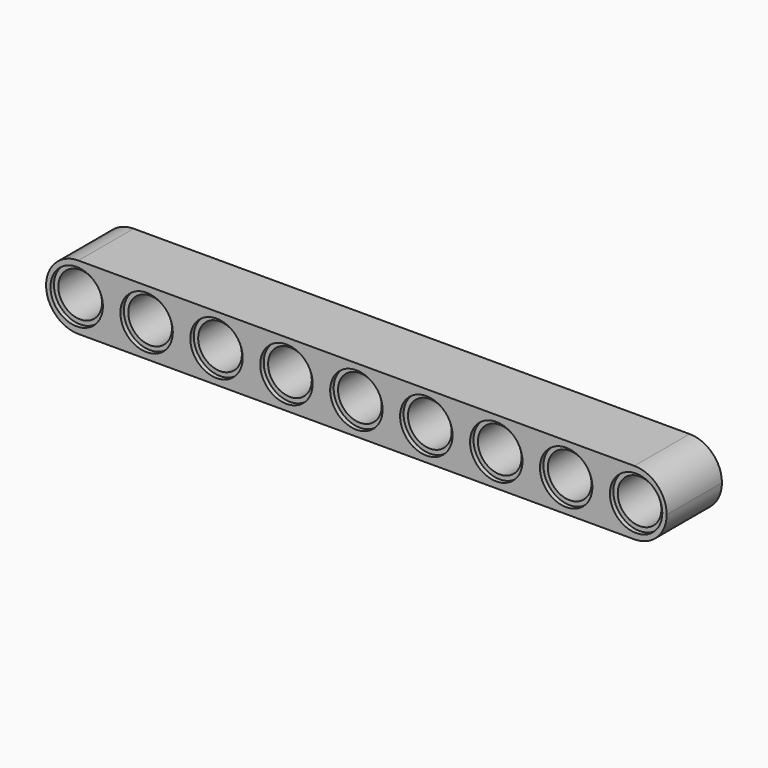
from build123d import *

# Parameters (mm, degrees)
F1_DEPTH = 3.95
F2_DEPTH = 3.45
F3_R     = 3.69999


# Not quite as in the source:
# - a fillet or chamfer is up to 0.001 mm smaller than in the source, because OpenCascade refuses the exact size


with BuildPart() as f1:
    # F0 (on Front) → F1 (new body, symmetric)
    with BuildSketch(Plane.XZ):
        with BuildLine():
            Line((21.3529593349, -11.1881163925), (-49.6470406651, -11.1881163925))
            Line((-49.6470406651, -11.1881163925), (-49.6470406651, -14.8881163925))
            Line((-49.6470406651, -14.8881163925), (-49.1470406651, -14.8881163925))
            ThreePointArc((-49.1470406651, -14.8881163925), (-46.1470406651, -11.8881163925), (-43.1470406651, -14.8881163925))
            Line((-43.1470406651, -14.8881163925), (-41.1470406651, -14.8881163925))
            ThreePointArc((-41.1470406651, -14.8881163925), (-38.1470406651, -11.8881163925), (-35.1470406651, -14.8881163925))
            Line((-35.1470406651, -14.8881163925), (-33.1470406651, -14.8881163925))
            ThreePointArc((-33.1470406651, -14.8881163925), (-30.1470406651, -11.8881163925), (-27.1470406651, -14.8881163925))
            Line((-27.1470406651, -14.8881163925), (-25.1470406651, -14.8881163925))
            ThreePointArc((-25.1470406651, -14.8881163925), (-22.1470406651, -11.8881163925), (-19.1470406651, -14.8881163925))
            Line((-19.1470406651, -14.8881163925), (-17.1470406651, -14.8881163925))
            ThreePointArc((-17.1470406651, -14.8881163925), (-14.1470406651, -11.8881163925), (-11.1470406651, -14.8881163925))
            Line((-11.1470406651, -14.8881163925), (-9.1470406651, -14.8881163925))
            ThreePointArc((-9.1470406651, -14.8881163925), (-6.1470406651, -11.8881163925), (-3.1470406651, -14.8881163925))
            Line((-3.1470406651, -14.8881163925), (-1.1470406651, -14.8881163925))
            ThreePointArc((-1.1470406651, -14.8881163925), (1.8529593349, -11.8881163925), (4.8529593349, -14.8881163925))
            Line((4.8529593349, -14.8881163925), (6.8529593349, -14.8881163925))
            ThreePointArc((6.8529593349, -14.8881163925), (9.8529593349, -11.8881163925), (12.8529593349, -14.8881163925))
            Line((12.8529593349, -14.8881163925), (14.8529593349, -14.8881163925))
            ThreePointArc((14.8529593349, -14.8881163925), (17.8529593349, -11.8881163925), (20.8529593349, -14.8881163925))
            Line((20.8529593349, -14.8881163925), (21.3529593349, -14.8881163925))
            Line((21.3529593349, -14.8881163925), (21.3529593349, -11.1881163925))
        make_face()
        with BuildLine():
            Line((-49.1470406651, -14.8881163925), (-49.6470406651, -14.8881163925))
            Line((-49.6470406651, -14.8881163925), (-49.6470406651, -18.5881163925))
            Line((-49.6470406651, -18.5881163925), (21.3529593349, -18.5881163925))
            Line((21.3529593349, -18.5881163925), (21.3529593349, -14.8881163925))
            Line((21.3529593349, -14.8881163925), (20.8529593349, -14.8881163925))
            ThreePointArc((20.8529593349, -14.8881163925), (17.8529593349, -17.8881163925), (14.8529593349, -14.8881163925))
            Line((14.8529593349, -14.8881163925), (12.8529593349, -14.8881163925))
            ThreePointArc((12.8529593349, -14.8881163925), (9.8529593349, -17.8881163925), (6.8529593349, -14.8881163925))
            Line((6.8529593349, -14.8881163925), (4.8529593349, -14.8881163925))
            ThreePointArc((4.8529593349, -14.8881163925), (1.8529593349, -17.8881163925), (-1.1470406651, -14.8881163925))
            Line((-1.1470406651, -14.8881163925), (-3.1470406651, -14.8881163925))
            ThreePointArc((-3.1470406651, -14.8881163925), (-6.1470406651, -17.8881163925), (-9.1470406651, -14.8881163925))
            Line((-9.1470406651, -14.8881163925), (-11.1470406651, -14.8881163925))
            ThreePointArc((-11.1470406651, -14.8881163925), (-14.1470406651, -17.8881163925), (-17.1470406651, -14.8881163925))
            Line((-17.1470406651, -14.8881163925), (-19.1470406651, -14.8881163925))
            ThreePointArc((-19.1470406651, -14.8881163925), (-22.1470406651, -17.8881163925), (-25.1470406651, -14.8881163925))
            Line((-25.1470406651, -14.8881163925), (-27.1470406651, -14.8881163925))
            ThreePointArc((-27.1470406651, -14.8881163925), (-30.1470406651, -17.8881163925), (-33.1470406651, -14.8881163925))
            Line((-33.1470406651, -14.8881163925), (-35.1470406651, -14.8881163925))
            ThreePointArc((-35.1470406651, -14.8881163925), (-38.1470406651, -17.8881163925), (-41.1470406651, -14.8881163925))
            Line((-41.1470406651, -14.8881163925), (-43.1470406651, -14.8881163925))
            ThreePointArc((-43.1470406651, -14.8881163925), (-46.1470406651, -17.8881163925), (-49.1470406651, -14.8881163925))
        make_face()
    extrude(amount=F1_DEPTH, both=True)

    # F0 (on Front) → F2 (join, symmetric)
    with BuildSketch(Plane.XZ):
        with BuildLine():
            ThreePointArc((-43.1470406651, -14.8881163925), (-46.1470406651, -11.8881163925), (-49.1470406651, -14.8881163925))
            Line((-49.1470406651, -14.8881163925), (-48.6470406651, -14.8881163925))
            ThreePointArc((-48.6470406651, -14.8881163925), (-46.1470406651, -12.3881163925), (-43.6470406651, -14.8881163925))
            Line((-43.6470406651, -14.8881163925), (-43.1470406651, -14.8881163925))
        make_face()
        with BuildLine():
            Line((-48.6470406651, -14.8881163925), (-49.1470406651, -14.8881163925))
            ThreePointArc((-49.1470406651, -14.8881163925), (-46.1470406651, -17.8881163925), (-43.1470406651, -14.8881163925))
            Line((-43.1470406651, -14.8881163925), (-43.6470406651, -14.8881163925))
            ThreePointArc((-43.6470406651, -14.8881163925), (-46.1470406651, -17.3881163925), (-48.6470406651, -14.8881163925))
        make_face()
        with BuildLine():
            ThreePointArc((14.8529593349, -14.8881163925), (17.8529593349, -17.8881163925), (20.8529593349, -14.8881163925))
            Line((20.8529593349, -14.8881163925), (20.3529593349, -14.8881163925))
            ThreePointArc((20.3529593349, -14.8881163925), (17.8529593349, -17.3881163925), (15.3529593349, -14.8881163925))
            Line((15.3529593349, -14.8881163925), (14.8529593349, -14.8881163925))
        make_face()
        with BuildLine():
            Line((20.3529593349, -14.8881163925), (20.8529593349, -14.8881163925))
            ThreePointArc((20.8529593349, -14.8881163925), (17.8529593349, -11.8881163925), (14.8529593349, -14.8881163925))
            Line((14.8529593349, -14.8881163925), (15.3529593349, -14.8881163925))
            ThreePointArc((15.3529593349, -14.8881163925), (17.8529593349, -12.3881163925), (20.3529593349, -14.8881163925))
        make_face()
        with BuildLine():
            ThreePointArc((-35.1470406651, -14.8881163925), (-38.1470406651, -11.8881163925), (-41.1470406651, -14.8881163925))
            Line((-41.1470406651, -14.8881163925), (-40.6470406651, -14.8881163925))
            ThreePointArc((-40.6470406651, -14.8881163925), (-38.1470406651, -12.3881163925), (-35.6470406651, -14.8881163925))
            Line((-35.6470406651, -14.8881163925), (-35.1470406651, -14.8881163925))
        make_face()
        with BuildLine():
            Line((-40.6470406651, -14.8881163925), (-41.1470406651, -14.8881163925))
            ThreePointArc((-41.1470406651, -14.8881163925), (-38.1470406651, -17.8881163925), (-35.1470406651, -14.8881163925))
            Line((-35.1470406651, -14.8881163925), (-35.6470406651, -14.8881163925))
            ThreePointArc((-35.6470406651, -14.8881163925), (-38.1470406651, -17.3881163925), (-40.6470406651, -14.8881163925))
        make_face()
        with BuildLine():
            ThreePointArc((6.8529593349, -14.8881163925), (9.8529593349, -17.8881163925), (12.8529593349, -14.8881163925))
            Line((12.8529593349, -14.8881163925), (12.3529593349, -14.8881163925))
            ThreePointArc((12.3529593349, -14.8881163925), (9.8529593349, -17.3881163925), (7.3529593349, -14.8881163925))
            Line((7.3529593349, -14.8881163925), (6.8529593349, -14.8881163925))
        make_face()
        with BuildLine():
            Line((12.3529593349, -14.8881163925), (12.8529593349, -14.8881163925))
            ThreePointArc((12.8529593349, -14.8881163925), (9.8529593349, -11.8881163925), (6.8529593349, -14.8881163925))
            Line((6.8529593349, -14.8881163925), (7.3529593349, -14.8881163925))
            ThreePointArc((7.3529593349, -14.8881163925), (9.8529593349, -12.3881163925), (12.3529593349, -14.8881163925))
        make_face()
        with BuildLine():
            ThreePointArc((-27.1470406651, -14.8881163925), (-30.1470406651, -11.8881163925), (-33.1470406651, -14.8881163925))
            Line((-33.1470406651, -14.8881163925), (-32.6470406651, -14.8881163925))
            ThreePointArc((-32.6470406651, -14.8881163925), (-30.1470406651, -12.3881163925), (-27.6470406651, -14.8881163925))
            Line((-27.6470406651, -14.8881163925), (-27.1470406651, -14.8881163925))
        make_face()
        with BuildLine():
            Line((-32.6470406651, -14.8881163925), (-33.1470406651, -14.8881163925))
            ThreePointArc((-33.1470406651, -14.8881163925), (-30.1470406651, -17.8881163925), (-27.1470406651, -14.8881163925))
            Line((-27.1470406651, -14.8881163925), (-27.6470406651, -14.8881163925))
            ThreePointArc((-27.6470406651, -14.8881163925), (-30.1470406651, -17.3881163925), (-32.6470406651, -14.8881163925))
        make_face()
        with BuildLine():
            ThreePointArc((-1.1470406651, -14.8881163925), (1.8529593349, -17.8881163925), (4.8529593349, -14.8881163925))
            Line((4.8529593349, -14.8881163925), (4.3529593349, -14.8881163925))
            ThreePointArc((4.3529593349, -14.8881163925), (1.8529593349, -17.3881163925), (-0.6470406651, -14.8881163925))
            Line((-0.6470406651, -14.8881163925), (-1.1470406651, -14.8881163925))
        make_face()
        with BuildLine():
            Line((4.3529593349, -14.8881163925), (4.8529593349, -14.8881163925))
            ThreePointArc((4.8529593349, -14.8881163925), (1.8529593349, -11.8881163925), (-1.1470406651, -14.8881163925))
            Line((-1.1470406651, -14.8881163925), (-0.6470406651, -14.8881163925))
            ThreePointArc((-0.6470406651, -14.8881163925), (1.8529593349, -12.3881163925), (4.3529593349, -14.8881163925))
        make_face()
        with BuildLine():
            ThreePointArc((-19.1470406651, -14.8881163925), (-22.1470406651, -11.8881163925), (-25.1470406651, -14.8881163925))
            Line((-25.1470406651, -14.8881163925), (-24.6470406651, -14.8881163925))
            ThreePointArc((-24.6470406651, -14.8881163925), (-22.1470406651, -12.3881163925), (-19.6470406651, -14.8881163925))
            Line((-19.6470406651, -14.8881163925), (-19.1470406651, -14.8881163925))
        make_face()
        with BuildLine():
            Line((-24.6470406651, -14.8881163925), (-25.1470406651, -14.8881163925))
            ThreePointArc((-25.1470406651, -14.8881163925), (-22.1470406651, -17.8881163925), (-19.1470406651, -14.8881163925))
            Line((-19.1470406651, -14.8881163925), (-19.6470406651, -14.8881163925))
            ThreePointArc((-19.6470406651, -14.8881163925), (-22.1470406651, -17.3881163925), (-24.6470406651, -14.8881163925))
        make_face()
        with BuildLine():
            ThreePointArc((-9.1470406651, -14.8881163925), (-6.1470406651, -17.8881163925), (-3.1470406651, -14.8881163925))
            Line((-3.1470406651, -14.8881163925), (-3.6470406651, -14.8881163925))
            ThreePointArc((-3.6470406651, -14.8881163925), (-6.1470406651, -17.3881163925), (-8.6470406651, -14.8881163925))
            Line((-8.6470406651, -14.8881163925), (-9.1470406651, -14.8881163925))
        make_face()
        with BuildLine():
            Line((-3.6470406651, -14.8881163925), (-3.1470406651, -14.8881163925))
            ThreePointArc((-3.1470406651, -14.8881163925), (-6.1470406651, -11.8881163925), (-9.1470406651, -14.8881163925))
            Line((-9.1470406651, -14.8881163925), (-8.6470406651, -14.8881163925))
            ThreePointArc((-8.6470406651, -14.8881163925), (-6.1470406651, -12.3881163925), (-3.6470406651, -14.8881163925))
        make_face()
        with BuildLine():
            ThreePointArc((-11.1470406651, -14.8881163925), (-14.1470406651, -11.8881163925), (-17.1470406651, -14.8881163925))
            Line((-17.1470406651, -14.8881163925), (-16.6470406651, -14.8881163925))
            ThreePointArc((-16.6470406651, -14.8881163925), (-14.1470406651, -12.3881163925), (-11.6470406651, -14.8881163925))
            Line((-11.6470406651, -14.8881163925), (-11.1470406651, -14.8881163925))
        make_face()
        with BuildLine():
            Line((-16.6470406651, -14.8881163925), (-17.1470406651, -14.8881163925))
            ThreePointArc((-17.1470406651, -14.8881163925), (-14.1470406651, -17.8881163925), (-11.1470406651, -14.8881163925))
            Line((-11.1470406651, -14.8881163925), (-11.6470406651, -14.8881163925))
            ThreePointArc((-11.6470406651, -14.8881163925), (-14.1470406651, -17.3881163925), (-16.6470406651, -14.8881163925))
        make_face()
    extrude(amount=F2_DEPTH, both=True)

    # F3 (radius 3.7 in the source; OpenCascade refuses exactly that, so slightly less here)
    f3_edges = [f1.edges().sort_by_distance(p)[0] for p in [
        (21.352959, 0, -11.188116),
        (21.352959, 0, -18.588116),
        (-49.647041, 0, -11.188116),
        (-49.647041, 0, -18.588116),
    ]]
    fillet(f3_edges, radius=F3_R)


solid = f1.part
